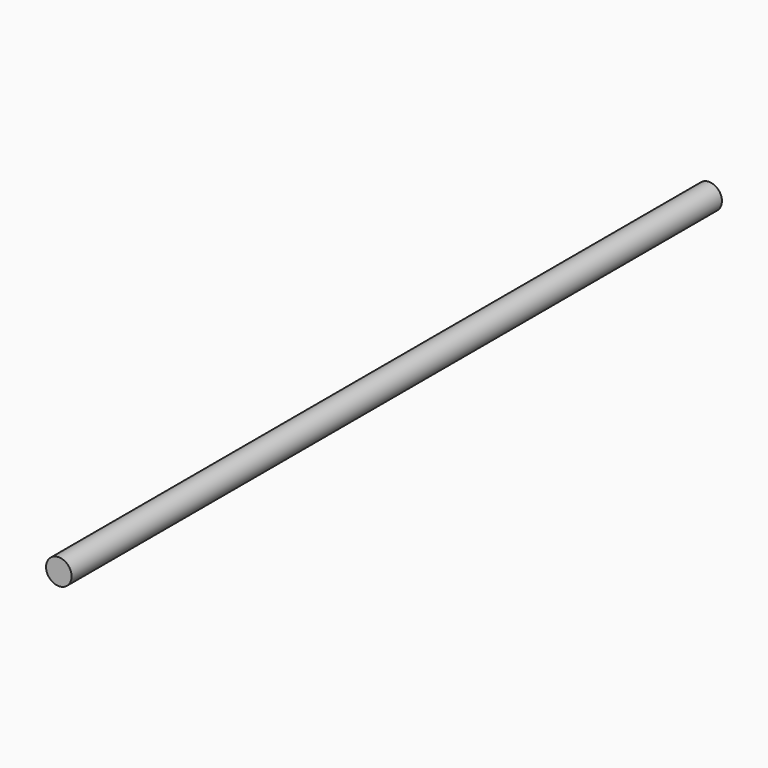
from build123d import *

# Parameters (mm, degrees)
F0_R     = 2.3510578695
F1_DEPTH = 149.86
F2_R     = 2.1421999077
F3_DEPTH = 12.7


# Not quite as in the source:
# - the program builds the solid bodies; features that only make, move or delete a surface that nothing else refers to are left out


with BuildPart() as f1:
    # F0 (on Front) → F1 (new body)
    with BuildSketch(Plane.XZ):
        with Locations((51.3897947967, 26.4229420573)):
            Circle(F0_R)
    extrude(amount=-F1_DEPTH)

    # F2 (on face) → F3 (cut)
    with BuildSketch(Plane(origin=(0, 149.86, 0), x_dir=(-1, 0, 0), z_dir=(0, 1, 0))):
        with Locations((-51.3897947967, 26.4229420573)):
            Circle(F2_R)
    extrude(amount=-F3_DEPTH, mode=Mode.SUBTRACT)


solid = f1.part
